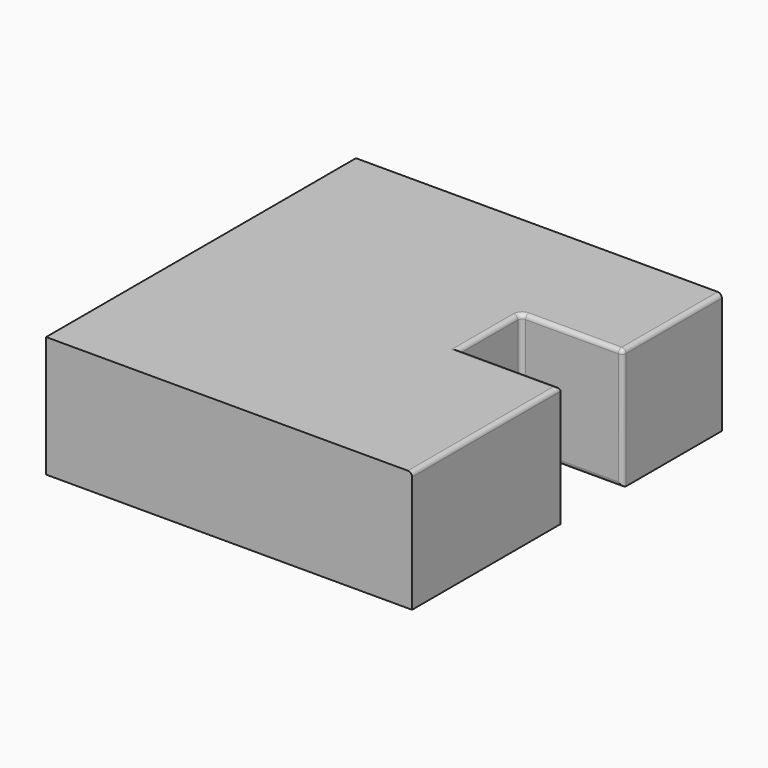
from build123d import *

# Parameters (mm, degrees)
F1_DEPTH = 15.3468120843
F2_R     = 0.540493976


with BuildPart() as f1:
    # F0 (on Top) → F1 (new body)
    with BuildSketch(Plane.XY):
        Polygon((-46.3772900403, 15.7230943441), (-46.3772900403, -33.35686028), (0, -33.35686028), (0, -9.8423212767), (-12.8479711711, -9.8423212767), (-12.8479711711, 0), (0, 0), (0, 15.7230943441), align=None)
    extrude(amount=F1_DEPTH)

    # F2
    f2_edges = [f1.edges().sort_by_distance(p)[0] for p in [
        (0, -21.599591, 15.346812),
        (0, 7.861547, 15.346812),
        (-12.847971, -4.921161, 15.346812),
        (-6.423986, -9.842321, 15.346812),
        (-12.847971, 0, 7.673406),
        (0, 0, 7.673406),
        (-6.423986, 0, 0),
        (-6.423986, 0, 15.346812),
        (-12.847971, -4.921161, 0),
    ]]
    fillet(f2_edges, radius=F2_R)


solid = f1.part
